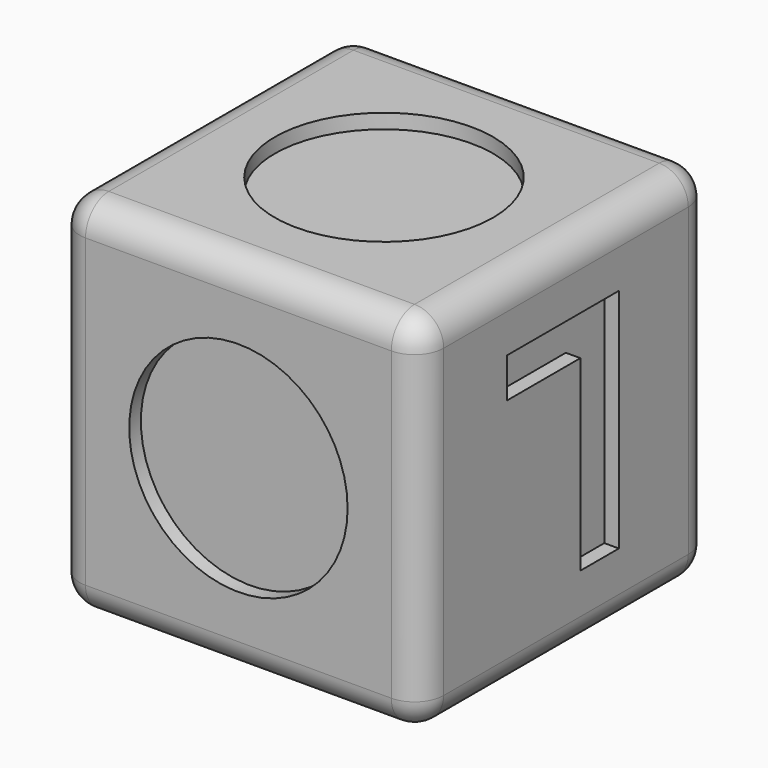
from build123d import *

# Parameters (mm, degrees)
F0_W          = 25
F0_H          = 25
F1_DEPTH      = 25
F2_R          = 7.5
F3_DEPTH      = 1
F4_R          = 7.5
F5_DEPTH      = 1
F6_R          = 7.5
F7_DEPTH      = 1
F8_TEXT_SIZE  = 21.8258132214
F9_DEPTH      = 1
F10_TEXT_SIZE = 20.6896551724
F11_DEPTH     = 1
F12_TEXT_SIZE = 22.4929709466
F13_DEPTH     = 1
F14_R         = 2


# Not quite as in the source:
# - Text() gives the source's letters only with a copy of the font that has no kerning and outlines rounded to 1/6400 em; it was checked with that copy


with BuildPart() as f1:
    # F0 (on Top) → F1 (new body)
    with BuildSketch(Plane.XY):
        Rectangle(F0_W, F0_H)
    extrude(amount=F1_DEPTH)

    # F2 (on face) → F3 (cut)
    with BuildSketch(Plane.XY.offset(25)):
        Circle(F2_R)
    extrude(amount=-F3_DEPTH, mode=Mode.SUBTRACT)

    # F4 (on face) → F5 (cut)
    with BuildSketch(Plane.XZ.offset(12.5)):
        with Locations((0, 12.5)):
            Circle(F4_R)
    extrude(amount=-F5_DEPTH, mode=Mode.SUBTRACT)

    # F6 (on face) → F7 (cut)
    with BuildSketch(Plane(origin=(0, 12.5, 0), x_dir=(-1, 0, 0), z_dir=(0, 1, 0))):
        with Locations((0, 12.5)):
            Circle(F6_R)
    extrude(amount=-F7_DEPTH, mode=Mode.SUBTRACT)

    # F8 (on face) → F9 (cut)
    with BuildSketch(Plane.YZ.offset(12.5)):
        with Locations(Location((6.5, 20.3572927597), (0, 0, 180))):
            Text('L', F8_TEXT_SIZE, font='Open Sans', font_style=FontStyle.BOLD, text_align=(TextAlign.LEFT, TextAlign.BOTTOM))
    extrude(amount=-F9_DEPTH, mode=Mode.SUBTRACT)

    # F10 (on face) → F11 (cut)
    with BuildSketch(Plane(origin=(-12.5, 0, 0), x_dir=(0, -1, 0), z_dir=(-1, 0, 0))):
        with Locations((-7.5, 5.0517241379)):
            Text('R', F10_TEXT_SIZE, font='Open Sans', font_style=FontStyle.BOLD, text_align=(TextAlign.LEFT, TextAlign.BOTTOM))
    extrude(amount=-F11_DEPTH, mode=Mode.SUBTRACT)

    # F12 (on face) → F13 (cut)
    with BuildSketch(Plane(origin=(0, 0, 0), x_dir=(1, 0, 0), z_dir=(0, 0, -1))):
        with Locations(Location((8.0974695408, -7.5), (0, 0, 90))):
            Text('C', F12_TEXT_SIZE, font='Open Sans', font_style=FontStyle.BOLD, text_align=(TextAlign.LEFT, TextAlign.BOTTOM))
    extrude(amount=-F13_DEPTH, mode=Mode.SUBTRACT)

    # F14
    f14_edges = [f1.edges().sort_by_distance(p)[0] for p in [
        (-12.5, 0, 0),
        (-12.5, 12.5, 12.5),
        (0, 12.5, 0),
        (0, 12.5, 25),
        (-12.5, 0, 25),
        (-12.5, -12.5, 12.5),
        (0, -12.5, 0),
        (12.5, -12.5, 12.5),
        (12.5, 0, 0),
        (12.5, 0, 25),
        (0, -12.5, 25),
        (12.5, 12.5, 12.5),
    ]]
    fillet(f14_edges, radius=F14_R)


solid = f1.part
